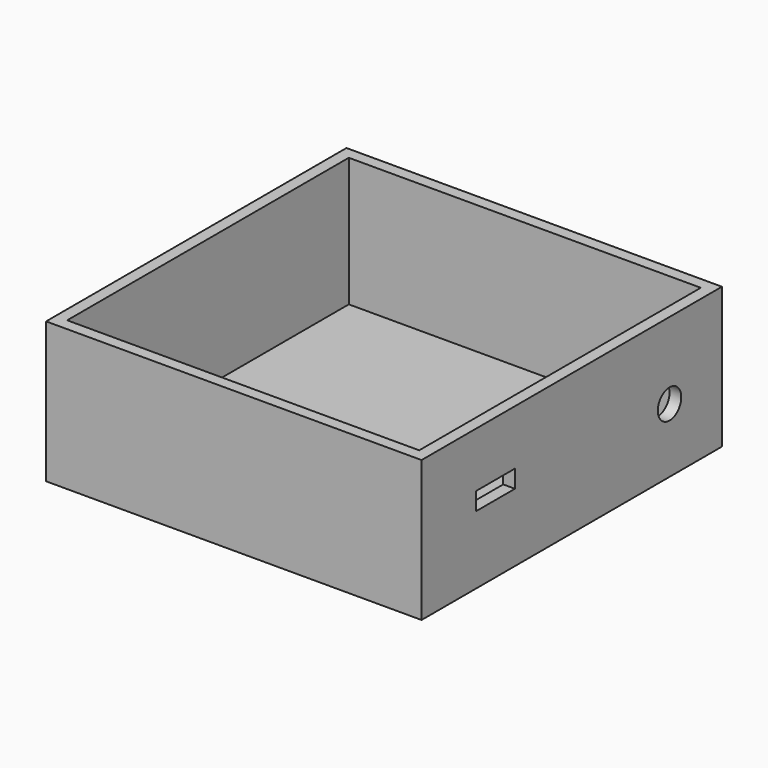
from build123d import *

# Parameters (mm, degrees)
F0_W     = 101.6
F0_H     = 38.1
F1_DEPTH = 101.6
F2_T     = -3.175
F4_D     = 7.9375
F4_DEPTH = 12.7
F4_TIP   = 2.3846655818
F3_W     = 13.1781175733
F3_H     = 4.8110592179
F5_DEPTH = 3.175


# Not quite as in the source:
# - a length typed as a fraction of an inch, garbled in the dataset ("3 / 203.2 mm" for 3/8 in), is restored


with BuildPart() as f1:
    # F0 (on Front) → F1 (new body)
    with BuildSketch(Plane.XZ):
        with Locations((10.0446864963, 7.5280469467)):
            Rectangle(F0_W, F0_H)
    extrude(amount=F1_DEPTH)

    # F2
    f2_openings = [f1.faces().sort_by_distance(p)[0] for p in [
        (10.044686, -50.8, 26.578047),
    ]]
    offset(amount=F2_T, openings=f2_openings)

    # F4
    with Locations(Plane.YZ.offset(60.8446864963)):
        with Locations((-17.720233649, 5.8569414541)):
            Hole(F4_D / 2, depth=F4_DEPTH)
            with Locations((0, 0, -(F4_DEPTH + F4_TIP / 2))):  # 118° drill point
                Cone(0, F4_D / 2, F4_TIP, mode=Mode.SUBTRACT)

    # F3 (on face) → F5 (cut, through all)
    with BuildSketch(Plane.YZ.offset(60.8446864963)):
        with Locations((-76.6034089029, 9.3083532993)):
            Rectangle(F3_W, F3_H)
    extrude(amount=-F5_DEPTH, mode=Mode.SUBTRACT)


solid = f1.part
